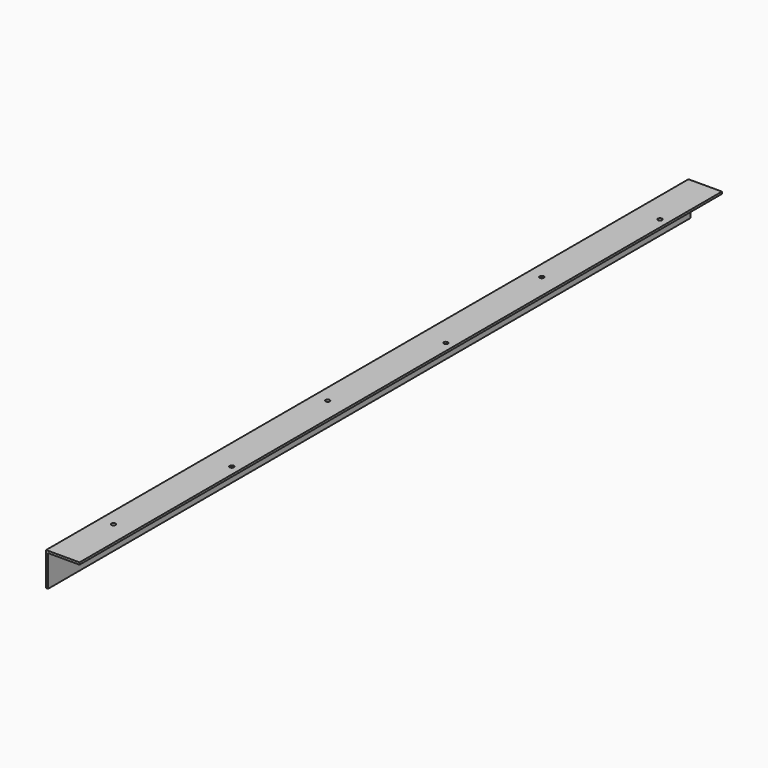
from build123d import *

# Parameters (mm, degrees)
F1_DEPTH = 1828.8
F3_D     = 12.7
F5_D     = 9.525
F6_ANGLE = 180
F9_D     = 7.9375


# Not quite as in the source:
# - a length typed as a fraction of an inch, garbled in the dataset ("3 / 203.2 mm" for 3/8 in), is restored
# - a feature names something its author has since deleted; it is built from what else it names


with BuildPart() as f1:
    # F0 (on Front) → F1 (new body)
    with BuildSketch(Plane.XZ):
        Polygon((-59.9026924796, 82.7025878191), (-59.9026924796, 6.5025878191), (16.2973075204, 6.5025878191), (16.2973075204, 11.2650878191), (-55.1401924796, 11.2650878191), (-55.1401924796, 82.7025878191), align=None)
    extrude(amount=F1_DEPTH)

    # F3 (through all)
    with Locations(Plane.YZ.offset(-55.1401924796)):
        with Locations((-203.2, 63.6525878191), (-1625.6, 63.6525878191)):
            Hole(F3_D / 2)

    # F5 (through all)
    with Locations(Plane(origin=(0, 0, 0), x_dir=(1, 0, 0), z_dir=(0, 0, -1))):
        with Locations((-28.1526924796, 1371.6), (-2.7526924796, 1676.4), (-2.7526924796, 1066.8), (-28.1526924796, 762), (-2.7526924796, 457.2), (-28.1526924796, 152.4)):
            Hole(F5_D / 2)


with BuildPart() as f1_1:
    # F6: moved
    add(f1.part.rotate(Axis((-19.4214424796, -1828.8, 11.2650878191), (-1, 0, 0)), F6_ANGLE))


with BuildPart() as f1_2:
    # F7: moved
    add(f1_1.part.moved(Location((0, 1828.8, 0))))

    # F9 (through all)
    with Locations(Plane.YZ.offset(-55.1401924796)):
        with Locations((-152.4, -1.4349121809), (-304.8, -1.4349121809), (-457.2, -1.4349121809), (-609.6, -1.4349121809), (-762, -1.4349121809), (-914.4, -1.4349121809), (-1066.8, -1.4349121809), (-1219.2, -1.4349121809), (-1371.6, -1.4349121809), (-1524, -1.4349121809), (-1676.4, -1.4349121809)):
            Hole(F9_D / 2)


solid = f1_2.part
